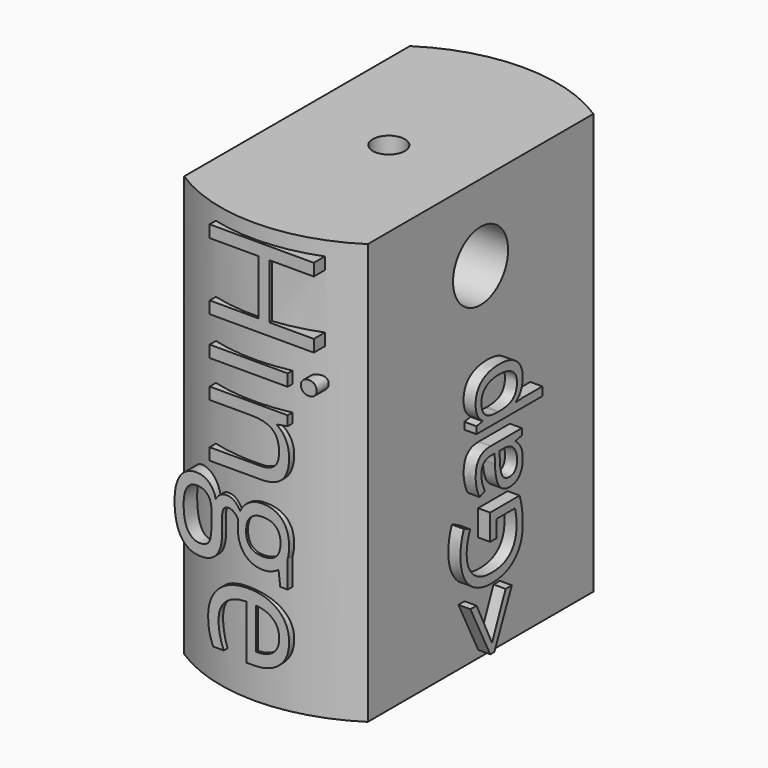
from build123d import *

# Parameters (mm, degrees)
F0_R          = 1.3335
F1_DEPTH      = 34.925
F2_R          = 2.8575
F3_DEPTH      = 7.62
F4_R          = 2.8575
F5_DEPTH      = 7.62
F6_TEXT_SIZE  = 8.8194444444
F7_DEPTH      = 1
F8_TEXT_SIZE  = 8.8194444444
F9_DEPTH      = 1
F11_TEXT_SIZE = 12.1132637854
F12_DEPTH     = 4


# Not quite as in the source:
# - Text() gives the source's letters only with a copy of the font that has no kerning and outlines rounded to 1/6400 em; it was checked with that copy


with BuildPart() as f1:
    # F0 (on Top) → F1 (new body)
    with BuildSketch(Plane.XY):
        with BuildLine():
            Line((-7.62, 11.7088214608), (-7.62, -11.7088214608))
            ThreePointArc((-7.62, -11.7088214608), (0, -13.97), (7.62, -11.7088214608))
            Line((7.62, -11.7088214608), (7.62, 11.7088214608))
            ThreePointArc((7.62, 11.7088214608), (0, 13.97), (-7.62, 11.7088214608))
        make_face()
        Circle(F0_R, mode=Mode.SUBTRACT)
    extrude(amount=F1_DEPTH)

    # F2 (on Right) → F3 (cut, through all)
    with BuildSketch(Plane.YZ):
        with Locations((0, 28.575)):
            Circle(F2_R)
    extrude(amount=F3_DEPTH, mode=Mode.SUBTRACT)

    # F4 (on Right) → F5 (cut, through all)
    with BuildSketch(Plane.YZ):
        with Locations((0, 6.35)):
            Circle(F4_R)
    extrude(amount=-F5_DEPTH, mode=Mode.SUBTRACT)

    # F6 (on face) → F7 (join)
    with BuildSketch(Plane(origin=(-7.62, 0, 0), x_dir=(0, -1, 0), z_dir=(-1, 0, 0))):
        with Locations(Location((3.7399669673, 30.3943946801), (0, 0, -90))):
            Text('<No', F6_TEXT_SIZE, font='Open Sans', text_align=(TextAlign.LEFT, TextAlign.BOTTOM))
        with Locations(Location((-8.2544774772, 28.1027171628), (0, 0, -90))):
            Text('Gap', F6_TEXT_SIZE, font='Open Sans', text_align=(TextAlign.LEFT, TextAlign.BOTTOM))
    extrude(amount=F7_DEPTH)

    # F8 (on face) → F9 (join)
    with BuildSketch(Plane.YZ.offset(7.62)):
        with Locations(Location((3.0399855273, 0.1541516324), (0, 0, 90))):
            Text('<Gap', F8_TEXT_SIZE, font='Open Sans', text_align=(TextAlign.LEFT, TextAlign.BOTTOM))
    extrude(amount=F9_DEPTH)

    # F11 (on offset) → F12 (join)
    with BuildSketch(Plane.XZ.offset(10.16)):
        with Locations(Location((-3.5492549302, 34.925), (0, 0, -90))):
            Text('Hinge', F11_TEXT_SIZE, font='Open Sans', text_align=(TextAlign.LEFT, TextAlign.BOTTOM))
    extrude(amount=F12_DEPTH)


solid = f1.part
